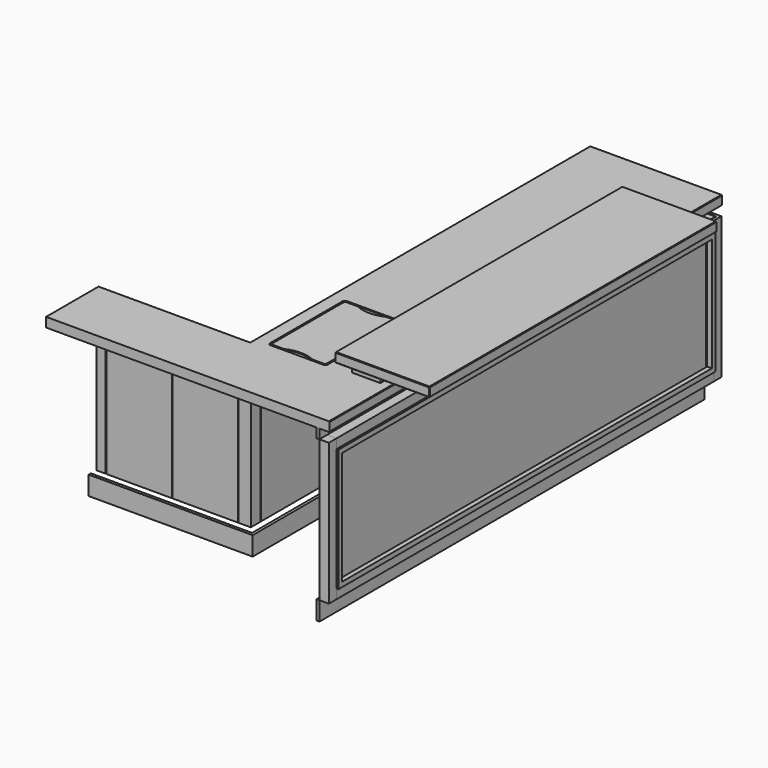
from build123d import *

# Parameters (mm, degrees)
F1_START       = 900
F0_W           = 350
F0_H           = 250
F1_DEPTH       = 50
F3_START       = 50
F2_W           = 250
F2_H           = 1900
F2_W_2         = 150
F2_H_2         = 150
F3_DEPTH       = 50
F4_DEPTH       = 50
F5_SIZE        = 3
F5_2_SIZE      = 3
F6_W           = 564
F6_H           = 15
F6_W_2         = 15
F6_H_2         = 2235
F6_W_3         = 278
F6_W_4         = 350
F6_W_5         = 225
F7_DEPTH       = 100
F8_START       = 100
F6_W_6         = 50
F8_DEPTH       = 750
F6_W_7         = 347
F6_H_3         = 50
F6_H_4         = 467.5
F6_H_5         = 600
F9_START       = 850
F9_DEPTH       = 50
F10_START      = 800
F10_DEPTH      = 50
F11_START      = 100
F6_W_8         = 35
F11_DEPTH      = 750
F6_W_9         = 588
F12_START      = 100
F12_DEPTH      = 750
F13_START      = 100
F13_DEPTH      = 750
F14_START      = 800
F14_DEPTH      = 50
F15_W          = 2497
F15_H          = 650
F15_W_2        = 2447
F15_H_2        = 600
F16_DEPTH      = 45
F17_DEPTH      = 10
F17_DEPTH_BACK = 15
F18_START      = -40
F18_DEPTH      = 5
F6_W_10        = 250
F6_H_6         = 450
F6_R           = 25
F6_W_11        = 200
F6_H_7         = 300
F19_DEPTH      = 1047
F20_START      = 900
F20_DEPTH      = 30
F21_START      = 930
F21_DEPTH      = 20
F22_R          = 13
F23_R          = 10
F24_SIZE       = 3
F24_2_SIZE     = 3


with BuildPart() as f1:
    # F0 (on Top) → F1 (new body)
    with BuildSketch(Plane.XY.offset(F1_START)):
        Polygon((0, 350), (0, 0), (1500, 0), (1500, 2600), (800, 2600), (800, 350), align=None)
        with Locations((400, 175)):
            Rectangle(F0_W, F0_H, mode=Mode.SUBTRACT)
        with Locations((400, 175)):
            Rectangle(F0_W, F0_H)
    extrude(amount=F1_DEPTH)

    # F5
    f5_edges = [f1.edges().sort_by_distance(p)[0] for p in [
        (1500, 2600, 925),
        (800, 2600, 925),
        (400, 350, 950),
        (800, 1475, 900),
        (800, 1475, 950),
        (400, 350, 900),
        (1150, 2600, 950),
        (1150, 2600, 900),
        (1500, 1300, 950),
        (1500, 1300, 900),
    ]]
    chamfer(f5_edges, length=F5_SIZE)

    # F6 (on face) → F19 (cut)
    with BuildSketch(Plane.XY):
        Polygon((1023, 883.75), (873, 883.75), (873, 383.75), (1173, 383.75), (1173, 633.75), (1170, 633.75), (1170, 386.75), (1098, 386.75), (948, 386.75), (876, 386.75), (876, 880.75), (948, 880.75), (1023, 880.75), align=None)
        with BuildLine():
            ThreePointArc((1023, 863.75), (984.5487321405, 868.0532300318), (948, 880.75))
            Line((948, 880.75), (876, 880.75))
            Line((876, 880.75), (876, 386.75))
            Line((876, 386.75), (948, 386.75))
            ThreePointArc((948, 386.75), (1023, 403.75), (1098, 386.75))
            Line((1098, 386.75), (1170, 386.75))
            Line((1170, 386.75), (1170, 633.75))
            Line((1170, 633.75), (1170, 880.75))
            Line((1170, 880.75), (1098, 880.75))
            ThreePointArc((1098, 880.75), (1061.4512678595, 868.0532300318), (1023, 863.75))
        make_face()
        with Locations((1023, 633.75)):
            Rectangle(F6_W_10, F6_H_6, mode=Mode.SUBTRACT)
        with Locations((1023, 633.75)):
            Rectangle(F6_W_10, F6_H_6)
        with Locations((1098, 471.25)):
            Circle(F6_R, mode=Mode.SUBTRACT)
        with Locations((1023, 683.75)):
            Rectangle(F6_W_11, F6_H_7, mode=Mode.SUBTRACT)
        with BuildLine():
            Line((948, 386.75), (1098, 386.75))
            ThreePointArc((1098, 386.75), (1023, 403.75), (948, 386.75))
        make_face()
        with Locations((1098, 471.25)):
            Circle(F6_R)
        Polygon((1173, 883.75), (1023, 883.75), (1023, 880.75), (1098, 880.75), (1170, 880.75), (1170, 633.75), (1173, 633.75), align=None)
        with BuildLine():
            Line((1098, 880.75), (1023, 880.75))
            Line((1023, 880.75), (1023, 863.75))
            ThreePointArc((1023, 863.75), (1061.4512678595, 868.0532300318), (1098, 880.75))
        make_face()
        with Locations((1023, 683.75)):
            Rectangle(F6_W_11, F6_H_7)
        with BuildLine():
            Line((1023, 863.75), (1023, 880.75))
            Line((1023, 880.75), (948, 880.75))
            ThreePointArc((948, 880.75), (984.5487321405, 868.0532300318), (1023, 863.75))
        make_face()
    extrude(amount=F19_DEPTH, mode=Mode.SUBTRACT)

    # F6 (on face) → F20 (join)
    with BuildSketch(Plane.XY.offset(F20_START)):
        with BuildLine():
            ThreePointArc((1023, 863.75), (984.5487321405, 868.0532300318), (948, 880.75))
            Line((948, 880.75), (876, 880.75))
            Line((876, 880.75), (876, 386.75))
            Line((876, 386.75), (948, 386.75))
            ThreePointArc((948, 386.75), (1023, 403.75), (1098, 386.75))
            Line((1098, 386.75), (1170, 386.75))
            Line((1170, 386.75), (1170, 633.75))
            Line((1170, 633.75), (1170, 880.75))
            Line((1170, 880.75), (1098, 880.75))
            ThreePointArc((1098, 880.75), (1061.4512678595, 868.0532300318), (1023, 863.75))
        make_face()
        with Locations((1023, 633.75)):
            Rectangle(F6_W_10, F6_H_6, mode=Mode.SUBTRACT)
        with BuildLine():
            Line((1023, 863.75), (1023, 880.75))
            Line((1023, 880.75), (948, 880.75))
            ThreePointArc((948, 880.75), (984.5487321405, 868.0532300318), (1023, 863.75))
        make_face()
        with BuildLine():
            Line((1098, 880.75), (1023, 880.75))
            Line((1023, 880.75), (1023, 863.75))
            ThreePointArc((1023, 863.75), (1061.4512678595, 868.0532300318), (1098, 880.75))
        make_face()
        with BuildLine():
            Line((948, 386.75), (1098, 386.75))
            ThreePointArc((1098, 386.75), (1023, 403.75), (948, 386.75))
        make_face()
        Polygon((1173, 883.75), (1023, 883.75), (1023, 880.75), (1098, 880.75), (1170, 880.75), (1170, 633.75), (1173, 633.75), align=None)
        Polygon((1023, 883.75), (873, 883.75), (873, 383.75), (1173, 383.75), (1173, 633.75), (1170, 633.75), (1170, 386.75), (1098, 386.75), (948, 386.75), (876, 386.75), (876, 880.75), (948, 880.75), (1023, 880.75), align=None)
    extrude(amount=F20_DEPTH)

    # F23
    f23_edges = [f1.edges().sort_by_distance(p)[0] for p in [
        (873, 383.75, 940),
        (873, 883.75, 940),
        (1173, 883.75, 940),
        (1173, 383.75, 940),
    ]]
    fillet(f23_edges, radius=F23_R)

    # F24
    f24_edges = [f1.edges().sort_by_distance(p)[0] for p in [
        (1023, 383.75, 950),
        (1170.071068, 386.678932, 950),
        (875.928932, 386.678932, 950),
        (1173, 633.75, 950),
        (873, 633.75, 950),
        (1170.071068, 880.821068, 950),
        (875.928932, 880.821068, 950),
        (1023, 883.75, 950),
    ]]
    chamfer(f24_edges, length=F24_SIZE)


with BuildPart() as f3:
    # F2 (on face) → F3 (new body)
    with BuildSketch(Plane.XY.offset(950).offset(F3_START)):
        with Locations((1625, 1300)):
            Rectangle(F2_W, F2_H)
        with Locations((1375, 1300)):
            Rectangle(F2_W, F2_H)
        with Locations((1375, 475)):
            Rectangle(F2_W_2, F2_H_2, mode=Mode.SUBTRACT)
        with Locations((1375, 1025)):
            Rectangle(F2_W_2, F2_H_2, mode=Mode.SUBTRACT)
        with Locations((1375, 1575)):
            Rectangle(F2_W_2, F2_H_2, mode=Mode.SUBTRACT)
        with Locations((1375, 2125)):
            Rectangle(F2_W_2, F2_H_2, mode=Mode.SUBTRACT)
        with Locations((1375, 2125)):
            Rectangle(F2_W_2, F2_H_2)
        with Locations((1375, 1575)):
            Rectangle(F2_W_2, F2_H_2)
        with Locations((1375, 1025)):
            Rectangle(F2_W_2, F2_H_2)
        with Locations((1375, 475)):
            Rectangle(F2_W_2, F2_H_2)
    extrude(amount=F3_DEPTH)

    # F5#2
    f5_2_edges = [f3.edges().sort_by_distance(p)[0] for p in [
        (1500, 2250, 1050),
        (1250, 1300, 1050),
        (1500, 350, 1050),
        (1750, 1300, 1050),
        (1500, 2250, 1000),
        (1250, 1300, 1000),
        (1500, 350, 1000),
        (1750, 1300, 1000),
        (1750, 2250, 1025),
        (1250, 2250, 1025),
        (1250, 350, 1025),
        (1750, 350, 1025),
    ]]
    chamfer(f5_2_edges, length=F5_2_SIZE)


with BuildPart() as f4:
    # F2 (on face) → F4 (new body)
    with BuildSketch(Plane.XY.offset(950)):
        with Locations((1375, 1575)):
            Rectangle(F2_W_2, F2_H_2)
    extrude(amount=F4_DEPTH)


with BuildPart() as f4b:
    # F2 (on face) → F4, piece 2 (new body)
    with BuildSketch(Plane.XY.offset(950)):
        with Locations((1375, 2125)):
            Rectangle(F2_W_2, F2_H_2)
    extrude(amount=F4_DEPTH)


with BuildPart() as f4c:
    # F2 (on face) → F4, piece 3 (new body)
    with BuildSketch(Plane.XY.offset(950)):
        with Locations((1375, 1025)):
            Rectangle(F2_W_2, F2_H_2)
    extrude(amount=F4_DEPTH)


with BuildPart() as f4d:
    # F2 (on face) → F4, piece 4 (new body)
    with BuildSketch(Plane.XY.offset(950)):
        with Locations((1375, 475)):
            Rectangle(F2_W_2, F2_H_2)
    extrude(amount=F4_DEPTH)


with BuildPart() as f7:
    # F6 (on face) → F7 (new body)
    with BuildSketch(Plane.XY):
        with Locations((1150, 2539.5)):
            Rectangle(F6_W, F6_H)
        Polygon((1432, 2532), (1432, 0), (1447, 0), (1447, 50), (1447, 2532), align=None)
        with Locations((1439.5, 2539.5)):
            Rectangle(F6_W_2, F6_H)
        with Locations((860.5, 1414.5)):
            Rectangle(F6_W_2, F6_H_2)
        with Locations((860.5, 2539.5)):
            Rectangle(F6_W_2, F6_H)
        with Locations((860.5, 289.5)):
            Rectangle(F6_W_2, F6_H)
        with Locations((714, 289.5)):
            Rectangle(F6_W_3, F6_H)
        with Locations((400, 289.5)):
            Rectangle(F6_W_4, F6_H)
        with Locations((112.5, 289.5)):
            Rectangle(F6_W_5, F6_H)
    extrude(amount=F7_DEPTH)


with BuildPart() as f8:
    # F6 (on face) → F8 (new body)
    with BuildSketch(Plane.XY.offset(F8_START)):
        with Locations((25, 339.5)):
            Rectangle(F6_W_6, F6_H)
    extrude(amount=F8_DEPTH)


with BuildPart() as f8b:
    # F6 (on face) → F8, piece 2 (new body)
    with BuildSketch(Plane.XY.offset(F8_START)):
        with Locations((226.5, 339.5)):
            Rectangle(F6_W_7, F6_H)
    extrude(amount=F8_DEPTH)


with BuildPart() as f8c:
    # F6 (on face) → F8, piece 3 (new body)
    with BuildSketch(Plane.XY.offset(F8_START)):
        with Locations((576.5, 339.5)):
            Rectangle(F6_W_7, F6_H)
    extrude(amount=F8_DEPTH)


with BuildPart() as f8d:
    # F6 (on face) → F8, piece 4 (new body)
    with BuildSketch(Plane.XY.offset(F8_START)):
        with Locations((778, 339.5)):
            Rectangle(F6_W_6, F6_H)
        with Locations((810.5, 339.5)):
            Rectangle(F6_W_2, F6_H)
        with Locations((810.5, 372)):
            Rectangle(F6_W_2, F6_H_3)
    extrude(amount=F8_DEPTH)


with BuildPart() as f8e:
    # F6 (on face) → F8, piece 5 (new body)
    with BuildSketch(Plane.XY.offset(F8_START)):
        with Locations((810.5, 633.75)):
            Rectangle(F6_W_2, F6_H_4)
    extrude(amount=F8_DEPTH)


with BuildPart() as f8f:
    # F6 (on face) → F8, piece 6 (new body)
    with BuildSketch(Plane.XY.offset(F8_START)):
        with Locations((810.5, 1170.5)):
            Rectangle(F6_W_2, F6_H_5)
    extrude(amount=F8_DEPTH)


with BuildPart() as f8g:
    # F6 (on face) → F8, piece 7 (new body)
    with BuildSketch(Plane.XY.offset(F8_START)):
        with Locations((810.5, 1773.5)):
            Rectangle(F6_W_2, F6_H_5)
    extrude(amount=F8_DEPTH)


with BuildPart() as f8h:
    # F6 (on face) → F8, piece 8 (new body)
    with BuildSketch(Plane.XY.offset(F8_START)):
        with Locations((810.5, 2310.25)):
            Rectangle(F6_W_2, F6_H_4)
    extrude(amount=F8_DEPTH)


with BuildPart() as f8i:
    # F6 (on face) → F8, piece 9 (new body)
    with BuildSketch(Plane.XY.offset(F8_START)):
        Polygon((803, 2547), (818, 2547), (818, 2582), (818, 2597), (803, 2597), align=None)
    extrude(amount=F8_DEPTH)

    # F6 (on face) → F11 (join)
    with BuildSketch(Plane.XY.offset(F11_START)):
        Polygon((803, 2547), (818, 2547), (818, 2582), (818, 2597), (803, 2597), align=None)
        with Locations((835.5, 2589.5)):
            Rectangle(F6_W_8, F6_H)
    extrude(amount=F11_DEPTH)


with BuildPart() as f9:
    # F6 (on face) → F9 (new body)
    with BuildSketch(Plane.XY.offset(F9_START)):
        with Locations((1150, 2539.5)):
            Rectangle(F6_W, F6_H)
        with Locations((1439.5, 2539.5)):
            Rectangle(F6_W_2, F6_H)
        Polygon((1432, 2532), (1432, 0), (1447, 0), (1447, 50), (1447, 2532), align=None)
        with Locations((860.5, 2539.5)):
            Rectangle(F6_W_2, F6_H)
        with Locations((860.5, 1414.5)):
            Rectangle(F6_W_2, F6_H_2)
        with Locations((860.5, 289.5)):
            Rectangle(F6_W_2, F6_H)
        with Locations((714, 289.5)):
            Rectangle(F6_W_3, F6_H)
        with Locations((400, 289.5)):
            Rectangle(F6_W_4, F6_H)
        with Locations((112.5, 289.5)):
            Rectangle(F6_W_5, F6_H)
    extrude(amount=F9_DEPTH)


with BuildPart() as f10:
    # F6 (on face) → F10 (new body)
    with BuildSketch(Plane.XY.offset(F10_START)):
        Polygon((753, 329), (0, 329), (0, 297), (225, 297), (225, 300), (575, 300), (575, 297), (853, 297), (853, 2532), (853, 2547), (821, 2547), (821, 397), (821, 329), align=None)
    extrude(amount=F10_DEPTH)


with BuildPart() as f11:
    # F6 (on face) → F11, piece 2 (new body)
    with BuildSketch(Plane.XY.offset(F11_START)):
        with Locations((1150, 2589.5)):
            Rectangle(F6_W_9, F6_H)
    extrude(amount=F11_DEPTH)


with BuildPart() as f11b:
    # F6 (on face) → F11, piece 3 (new body)
    with BuildSketch(Plane.XY.offset(F11_START)):
        Polygon((1447, 2597), (1447, 2582), (1482, 2582), (1482, 2547), (1497, 2547), (1497, 2597), align=None)
    extrude(amount=F11_DEPTH)


with BuildPart() as f12:
    # F6 (on face) → F12 (new body)
    with BuildSketch(Plane.XY.offset(F12_START)):
        Polygon((1447, 2532), (1447, 50), (1482, 50), (1497, 50), (1497, 2547), (1482, 2547), (1479, 2547), (1447, 2547), align=None)
    extrude(amount=F12_DEPTH)

    # F15 (on face) → F16 (cut)
    with BuildSketch(Plane.YZ.offset(1497)):
        with Locations((1298.5, 475)):
            Rectangle(F15_W, F15_H)
        with Locations((1298.5, 475)):
            Rectangle(F15_W_2, F15_H_2, mode=Mode.SUBTRACT)
        with Locations((1298.5, 475)):
            Rectangle(F15_W_2, F15_H_2)
    extrude(amount=-F16_DEPTH, mode=Mode.SUBTRACT)


with BuildPart() as f13:
    # F6 (on face) → F13 (new body)
    with BuildSketch(Plane.XY.offset(F13_START)):
        with Locations((1464.5, 25)):
            Rectangle(F6_W_8, F6_H_3)
        with Locations((1489.5, 25)):
            Rectangle(F6_W_2, F6_H_3)
    extrude(amount=F13_DEPTH)


with BuildPart() as f14:
    # F6 (on face) → F14 (new body)
    with BuildSketch(Plane.XY.offset(F14_START)):
        Polygon((821, 2579), (821, 2547), (853, 2547), (868, 2547), (1432, 2547), (1447, 2547), (1479, 2547), (1479, 2579), (1447, 2579), align=None)
    extrude(amount=F14_DEPTH)


with BuildPart() as f17:
    # F15 (on face) → F17 (new body, two sides)
    with BuildSketch(Plane.YZ.offset(1497)) as f17_sk:
        with Locations((1298.5, 475)):
            Rectangle(F15_W, F15_H)
        with Locations((1298.5, 475)):
            Rectangle(F15_W_2, F15_H_2, mode=Mode.SUBTRACT)
    extrude(amount=F17_DEPTH)
    extrude(f17_sk.sketch, amount=-F17_DEPTH_BACK)


with BuildPart() as f18:
    # F15 (on face) → F18 (new body)
    with BuildSketch(Plane.YZ.offset(1497).offset(F18_START)):
        with Locations((1298.5, 475)):
            Rectangle(F15_W, F15_H)
        with Locations((1298.5, 475)):
            Rectangle(F15_W_2, F15_H_2, mode=Mode.SUBTRACT)
        with Locations((1298.5, 475)):
            Rectangle(F15_W_2, F15_H_2)
    extrude(amount=-F18_DEPTH)


with BuildPart() as f21:
    # F6 (on face) → F21 (new body)
    with BuildSketch(Plane.XY.offset(F21_START)):
        with BuildLine():
            ThreePointArc((1023, 863.75), (984.5487321405, 868.0532300318), (948, 880.75))
            Line((948, 880.75), (876, 880.75))
            Line((876, 880.75), (876, 386.75))
            Line((876, 386.75), (948, 386.75))
            ThreePointArc((948, 386.75), (1023, 403.75), (1098, 386.75))
            Line((1098, 386.75), (1170, 386.75))
            Line((1170, 386.75), (1170, 633.75))
            Line((1170, 633.75), (1170, 880.75))
            Line((1170, 880.75), (1098, 880.75))
            ThreePointArc((1098, 880.75), (1061.4512678595, 868.0532300318), (1023, 863.75))
        make_face()
        with Locations((1023, 633.75)):
            Rectangle(F6_W_10, F6_H_6, mode=Mode.SUBTRACT)
        with Locations((1023, 633.75)):
            Rectangle(F6_W_10, F6_H_6)
        with Locations((1098, 471.25)):
            Circle(F6_R, mode=Mode.SUBTRACT)
        with Locations((1023, 683.75)):
            Rectangle(F6_W_11, F6_H_7, mode=Mode.SUBTRACT)
        with Locations((1023, 683.75)):
            Rectangle(F6_W_11, F6_H_7)
        with Locations((1098, 471.25)):
            Circle(F6_R)
    extrude(amount=F21_DEPTH)

    # F22
    f22_edges = [f21.edges().sort_by_distance(p)[0] for p in [
        (876, 880.75, 940),
        (876, 386.75, 940),
        (1098, 386.75, 940),
        (1098, 880.75, 940),
        (948, 386.75, 940),
        (1170, 386.75, 940),
        (1170, 880.75, 940),
        (948, 880.75, 940),
    ]]
    fillet(f22_edges, radius=F22_R)

    # F24#2
    f24_2_edges = [f21.edges().sort_by_distance(p)[0] for p in [
        (1128.945475, 386.75, 950),
        (1098.118904, 387.048986, 950),
        (1166.192388, 390.557612, 950),
        (1023, 403.75, 950),
        (1170, 633.75, 950),
        (947.881096, 387.048986, 950),
        (1166.192388, 876.942388, 950),
        (917.054525, 386.75, 950),
        (1128.945475, 880.75, 950),
        (879.807612, 390.557612, 950),
        (1098.118904, 880.451014, 950),
        (876, 633.75, 950),
        (1023, 863.75, 950),
        (879.807612, 876.942388, 950),
        (947.881096, 880.451014, 950),
        (917.054525, 880.75, 950),
    ]]
    chamfer(f24_2_edges, length=F24_2_SIZE)


solid = Compound([f1.part, f3.part, f4.part, f4b.part, f4c.part, f4d.part, f7.part, f8.part, f8b.part, f8c.part, f8d.part, f8e.part, f8f.part, f8g.part, f8h.part, f8i.part, f9.part, f10.part, f11.part, f11b.part, f12.part, f13.part, f14.part, f17.part, f18.part, f21.part])
